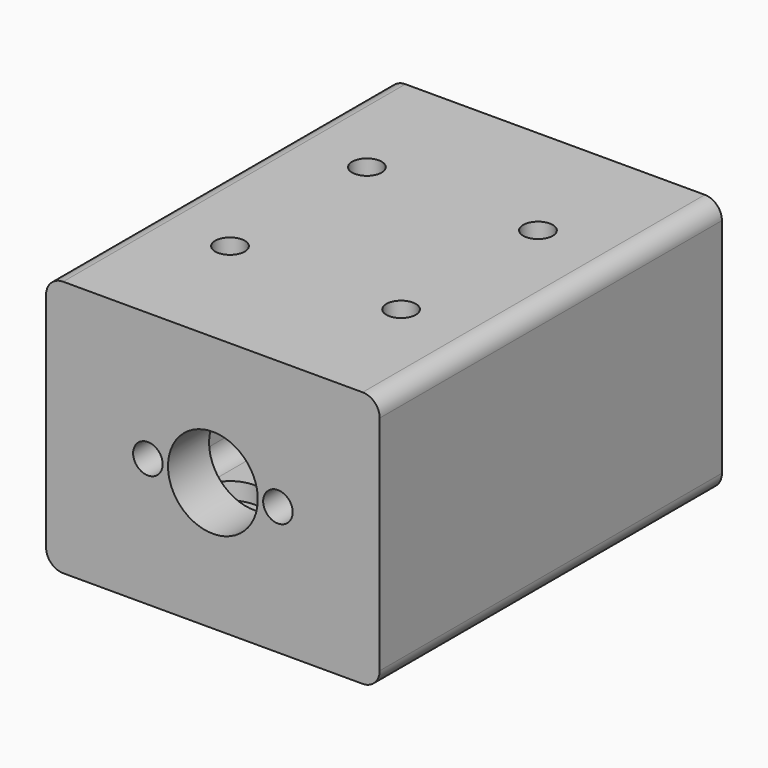
from build123d import *

# Parameters (mm, degrees)
F0_W      = 39
F0_H      = 50
F0_R      = 3.5
F0_R_2    = 1.725
F1_DEPTH  = 4
F2_R      = 3.5
F3_DEPTH  = 2
F5_DEPTH  = 22
F6_R      = 5.25
F6_R_2    = 1.725
F7_DEPTH  = 6
F8_W      = 39
F8_H      = 50
F9_DEPTH  = 4
F10_R     = 1.99999
F11_R     = 1.725
F12_DEPTH = 4
F14_DEPTH = 2


# Not quite as in the source:
# - a fillet or chamfer is up to 0.001 mm smaller than in the source, because OpenCascade refuses the exact size


with BuildPart() as f1:
    # F0 (on Top) → F1 (new body)
    with BuildSketch(Plane.XY):
        with Locations((19.5, 25)):
            Rectangle(F0_W, F0_H)
        with Locations((9.5, 15)):
            Circle(F0_R, mode=Mode.SUBTRACT)
        with Locations((29.5, 15)):
            Circle(F0_R, mode=Mode.SUBTRACT)
        with Locations((9.5, 35)):
            Circle(F0_R, mode=Mode.SUBTRACT)
        with Locations((29.5, 35)):
            Circle(F0_R, mode=Mode.SUBTRACT)
        with Locations((9.5, 35)):
            Circle(F0_R)
        with Locations((9.5, 35)):
            Circle(F0_R_2, mode=Mode.SUBTRACT)
        with Locations((29.5, 35)):
            Circle(F0_R)
        with Locations((29.5, 35)):
            Circle(F0_R_2, mode=Mode.SUBTRACT)
        with Locations((29.5, 15)):
            Circle(F0_R)
        with Locations((29.5, 15)):
            Circle(F0_R_2, mode=Mode.SUBTRACT)
        with Locations((9.5, 15)):
            Circle(F0_R)
        with Locations((9.5, 15)):
            Circle(F0_R_2, mode=Mode.SUBTRACT)
    extrude(amount=F1_DEPTH)

    # F2 (on face) → F3 (cut)
    with BuildSketch(Plane.XY.offset(4)):
        with Locations((9.5, 35)):
            Circle(F2_R)
        with Locations((29.5, 35)):
            Circle(F2_R)
        with Locations((29.5, 15)):
            Circle(F2_R)
        with Locations((9.5, 15)):
            Circle(F2_R)
    extrude(amount=-F3_DEPTH, mode=Mode.SUBTRACT)

    # F4 (on face) → F5 (join)
    with BuildSketch(Plane.XY.offset(4)):
        Polygon((4, 50), (0, 50), (0, 0), (39, 0), (39, 50), (35, 50), (35, 6), (4, 6), align=None)
    extrude(amount=F5_DEPTH)

    # F6 (on face) → F7 (cut, through all)
    with BuildSketch(Plane(origin=(0, 6, 0), x_dir=(-1, 0, 0), z_dir=(0, 1, 0))):
        with Locations((-19.5, 15)):
            Circle(F6_R)
        with Locations((-27.1, 15)):
            Circle(F6_R_2)
        with Locations((-11.9, 15)):
            Circle(F6_R_2)
    extrude(amount=-F7_DEPTH, mode=Mode.SUBTRACT)

    # F8 (on face) → F9 (join)
    with BuildSketch(Plane.XY.offset(26)):
        with Locations((19.5, 25)):
            Rectangle(F8_W, F8_H)
    extrude(amount=F9_DEPTH)

    # F10 (radius 2 in the source; OpenCascade refuses exactly that, so slightly less here)
    f10_edges = [f1.edges().sort_by_distance(p)[0] for p in [
        (0, 25, 30),
        (0, 25, 0),
        (39, 25, 0),
        (39, 25, 30),
        (35, 28, 26),
        (4, 28, 26),
        (4, 28, 4),
        (35, 28, 4),
    ]]
    fillet(f10_edges, radius=F10_R)

    # F11 (on face) → F12 (cut, through all)
    with BuildSketch(Plane.XY.offset(30)):
        with Locations((9.5, 35)):
            Circle(F11_R)
        with Locations((29.5, 35)):
            Circle(F11_R)
        with Locations((29.5, 15)):
            Circle(F11_R)
        with Locations((9.5, 15)):
            Circle(F11_R)
    extrude(amount=-F12_DEPTH, mode=Mode.SUBTRACT)

    # F13 (on face) → F14 (cut)
    with BuildSketch(Plane(origin=(0, 0, 26), x_dir=(1, 0, 0), z_dir=(0, 0, -1))):
        Polygon((12.26, -13.406513257), (9.5, -11.8130265141), (6.74, -13.406513257), (6.74, -16.593486743), (9.5, -18.1869734859), (12.26, -16.593486743), align=None)
        Polygon((32.26, -13.406513257), (29.5, -11.8130265141), (26.74, -13.406513257), (26.74, -16.593486743), (29.5, -18.1869734859), (32.26, -16.593486743), align=None)
        Polygon((32.26, -33.406513257), (29.5, -31.8130265141), (26.74, -33.406513257), (26.74, -36.593486743), (29.5, -38.1869734859), (32.26, -36.593486743), align=None)
        Polygon((12.26, -33.406513257), (9.5, -31.8130265141), (6.74, -33.406513257), (6.74, -36.593486743), (9.5, -38.1869734859), (12.26, -36.593486743), align=None)
    extrude(amount=-F14_DEPTH, mode=Mode.SUBTRACT)


solid = f1.part
